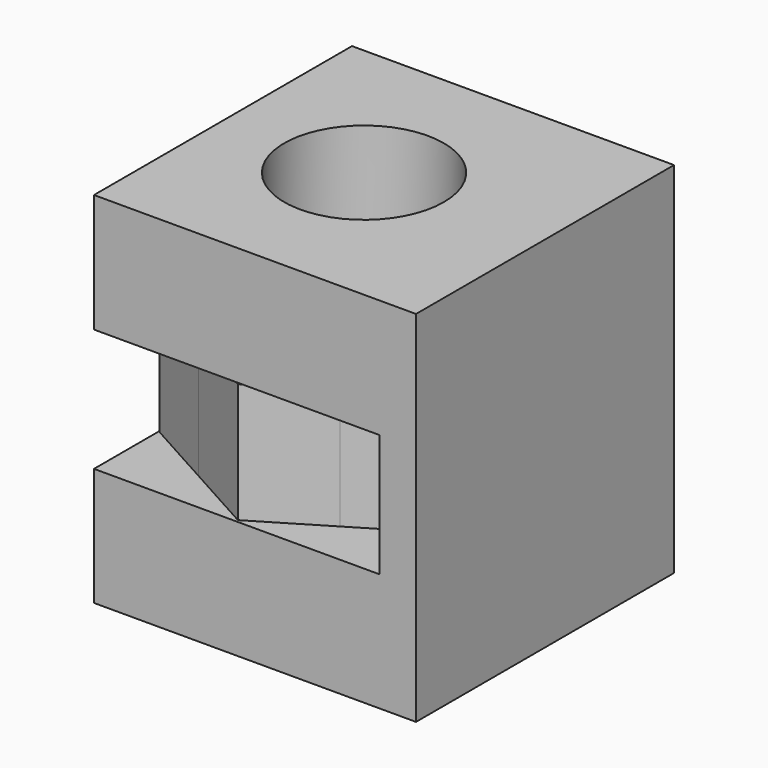
from build123d import *

# Parameters (mm, degrees)
F1_START = 3
F0_R     = 2
F1_DEPTH = 3
F2_DEPTH = 9
F3_W     = 7.1511580269
F3_H     = 3.0721682124
F4_DEPTH = 25


with BuildPart() as f1:
    # F0 (on Top) → F1 (new body)
    with BuildSketch(Plane.XY.offset(F1_START)):
        with BuildLine():
            ThreePointArc((-39.6189296859, 15.4045963577), (-39.1808945494, 17.1625789331), (-37.9225537154, 18.4660189438))
            Line((-37.9225537154, 18.4660189438), (-39.6544984202, 17.4250089553))
            Line((-39.6544984202, 17.4250089553), (-39.6189296859, 15.4045963577))
        make_face()
        with BuildLine():
            Line((-39.5833609418, 13.3841831991), (-37.8158476605, 12.4047801734))
            ThreePointArc((-37.8158476605, 12.4047801734), (-39.1192878718, 13.6631210573), (-39.6189296859, 15.4045963577))
            Line((-39.6189296859, 15.4045963577), (-39.5833609418, 13.3841831991))
        make_face()
        with BuildLine():
            Line((-36.0483344454, 11.4253771844), (-34.3163899469, 12.4663870488))
            ThreePointArc((-34.3163899469, 12.4663870488), (-36.0578650476, 11.9667451837), (-37.8158476605, 12.4047801734))
            Line((-37.8158476605, 12.4047801734), (-36.0483344454, 11.4253771844))
        make_face()
        with BuildLine():
            ThreePointArc((-32.6200141688, 15.5278099302), (-32.6196074877, 15.4970076286), (-32.6194719238, 15.4662029406))
            ThreePointArc((-32.6194719238, 15.4662029406), (-33.0730981024, 13.7429483046), (-34.3163899469, 12.4663870488))
            Line((-34.3163899469, 12.4663870488), (-32.5844454274, 13.5073969259))
            Line((-32.5844454274, 13.5073969259), (-32.6200141688, 15.5278099302))
        make_face()
        with BuildLine():
            ThreePointArc((-34.4230959253, 18.5276255628), (-33.1196560035, 17.26928487), (-32.6200141688, 15.5278099302))
            Line((-32.6200141688, 15.5278099302), (-32.6555829058, 17.5482226822))
            Line((-32.6555829058, 17.5482226822), (-34.4230959253, 18.5276255628))
        make_face()
        with BuildLine():
            ThreePointArc((-37.9225537154, 18.4660189438), (-36.1810785423, 18.9656607021), (-34.4230959253, 18.5276255628))
            Line((-34.4230959253, 18.5276255628), (-36.1906094022, 19.5070286969))
            Line((-36.1906094022, 19.5070286969), (-37.9225537154, 18.4660189438))
        make_face()
        with BuildLine():
            ThreePointArc((-34.3163899469, 12.4663870488), (-33.0730981024, 13.7429483046), (-32.6194719238, 15.4662029406))
            ThreePointArc((-32.6194719238, 15.4662029406), (-32.6196074877, 15.4970076286), (-32.6200141688, 15.5278099302))
            ThreePointArc((-32.6200141688, 15.5278099302), (-33.1196560035, 17.26928487), (-34.4230959253, 18.5276255628))
            ThreePointArc((-34.4230959253, 18.5276255628), (-36.1810785423, 18.9656607021), (-37.9225537154, 18.4660189438))
            ThreePointArc((-37.9225537154, 18.4660189438), (-39.1808945494, 17.1625789331), (-39.6189296859, 15.4045963577))
            ThreePointArc((-39.6189296859, 15.4045963577), (-39.1192878718, 13.6631210573), (-37.8158476605, 12.4047801734))
            ThreePointArc((-37.8158476605, 12.4047801734), (-36.0578650476, 11.9667451837), (-34.3163899469, 12.4663870488))
        make_face()
        with Locations((-36.1194719238, 15.4662029406)):
            Circle(F0_R, mode=Mode.SUBTRACT)
    extrude(amount=F1_DEPTH)


with BuildPart() as f2:
    # F0 (on Top) → F2 (new body)
    with BuildSketch(Plane.XY):
        with BuildLine():
            ThreePointArc((-39.6189296859, 15.4045963577), (-39.1808945494, 17.1625789331), (-37.9225537154, 18.4660189438))
            Line((-37.9225537154, 18.4660189438), (-39.6544984202, 17.4250089553))
            Line((-39.6544984202, 17.4250089553), (-39.6189296859, 15.4045963577))
        make_face()
        Polygon((-36.0483344454, 11.4253771844), (-37.8158476605, 12.4047801734), (-39.5833609418, 13.3841831991), (-39.6189296859, 15.4045963577), (-39.6544984202, 17.4250089553), (-39.6544984202, 11.4253771844), align=None)
        Polygon((-32.5844454274, 13.5073969259), (-34.3163899469, 12.4663870488), (-36.0483344454, 11.4253771844), (-32.5844454274, 11.4253771844), align=None)
        with BuildLine():
            ThreePointArc((-34.3163899469, 12.4663870488), (-33.0730981024, 13.7429483046), (-32.6194719238, 15.4662029406))
            ThreePointArc((-32.6194719238, 15.4662029406), (-32.6196074877, 15.4970076286), (-32.6200141688, 15.5278099302))
            ThreePointArc((-32.6200141688, 15.5278099302), (-33.1196560035, 17.26928487), (-34.4230959253, 18.5276255628))
            ThreePointArc((-34.4230959253, 18.5276255628), (-36.1810785423, 18.9656607021), (-37.9225537154, 18.4660189438))
            ThreePointArc((-37.9225537154, 18.4660189438), (-39.1808945494, 17.1625789331), (-39.6189296859, 15.4045963577))
            ThreePointArc((-39.6189296859, 15.4045963577), (-39.1192878718, 13.6631210573), (-37.8158476605, 12.4047801734))
            ThreePointArc((-37.8158476605, 12.4047801734), (-36.0578650476, 11.9667451837), (-34.3163899469, 12.4663870488))
        make_face()
        with Locations((-36.1194719238, 15.4662029406)):
            Circle(F0_R, mode=Mode.SUBTRACT)
        with BuildLine():
            ThreePointArc((-32.6200141688, 15.5278099302), (-32.6196074877, 15.4970076286), (-32.6194719238, 15.4662029406))
            ThreePointArc((-32.6194719238, 15.4662029406), (-33.0730981024, 13.7429483046), (-34.3163899469, 12.4663870488))
            Line((-34.3163899469, 12.4663870488), (-32.5844454274, 13.5073969259))
            Line((-32.5844454274, 13.5073969259), (-32.6200141688, 15.5278099302))
        make_face()
        Polygon((-39.6544984202, 17.4250089553), (-37.9225537154, 18.4660189438), (-36.1906094022, 19.5070286969), (-39.6544984202, 19.5070286969), align=None)
        Polygon((-32.5844454274, 19.5070286969), (-32.5844454274, 13.5073969259), (-32.5844454274, 11.4253771844), (-31.5844454274, 11.4253771844), (-31.5844454274, 19.5070286969), align=None)
        with BuildLine():
            ThreePointArc((-37.9225537154, 18.4660189438), (-36.1810785423, 18.9656607021), (-34.4230959253, 18.5276255628))
            Line((-34.4230959253, 18.5276255628), (-36.1906094022, 19.5070286969))
            Line((-36.1906094022, 19.5070286969), (-37.9225537154, 18.4660189438))
        make_face()
        Polygon((-32.6555829058, 17.5482226822), (-32.6200141688, 15.5278099302), (-32.5844454274, 13.5073969259), (-32.5844454274, 19.5070286969), (-36.1906094022, 19.5070286969), (-34.4230959253, 18.5276255628), align=None)
        with BuildLine():
            Line((-36.0483344454, 11.4253771844), (-34.3163899469, 12.4663870488))
            ThreePointArc((-34.3163899469, 12.4663870488), (-36.0578650476, 11.9667451837), (-37.8158476605, 12.4047801734))
            Line((-37.8158476605, 12.4047801734), (-36.0483344454, 11.4253771844))
        make_face()
        with BuildLine():
            Line((-39.5833609418, 13.3841831991), (-37.8158476605, 12.4047801734))
            ThreePointArc((-37.8158476605, 12.4047801734), (-39.1192878718, 13.6631210573), (-39.6189296859, 15.4045963577))
            Line((-39.6189296859, 15.4045963577), (-39.5833609418, 13.3841831991))
        make_face()
        with BuildLine():
            ThreePointArc((-34.4230959253, 18.5276255628), (-33.1196560035, 17.26928487), (-32.6200141688, 15.5278099302))
            Line((-32.6200141688, 15.5278099302), (-32.6555829058, 17.5482226822))
            Line((-32.6555829058, 17.5482226822), (-34.4230959253, 18.5276255628))
        make_face()
    extrude(amount=F2_DEPTH)

    # F3 (on face) → F4 (cut)
    with BuildSketch(Plane.XZ.offset(-11.4253771844)):
        with Locations((-36.0789194067, 4.4949187431)):
            Rectangle(F3_W, F3_H)
    extrude(amount=-F4_DEPTH, mode=Mode.SUBTRACT)


solid = Compound([f1.part, f2.part])
